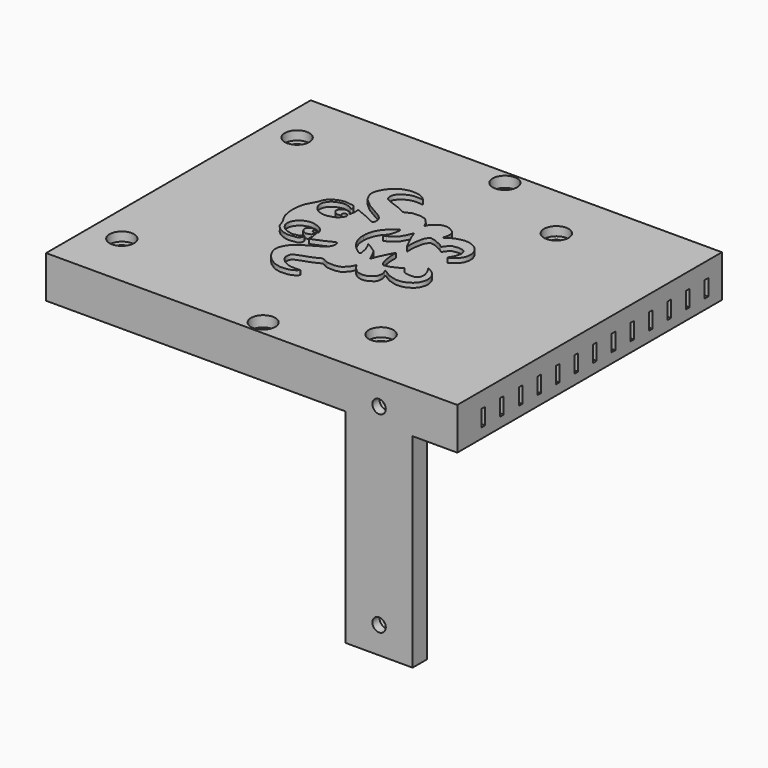
from build123d import *

# Parameters (mm, degrees)
F0_R      = 3
F0_R_2    = 1.45
F1_DEPTH  = 5
F2_W      = 88
F2_H      = 66
F3_DEPTH  = 3
F4_DEPTH  = 25
F5_R      = 2.75
F6_DEPTH  = 2
F7_W      = 7
F7_H      = 2
F8_DEPTH  = 9.4
F9_W      = 22.6646959782
F9_H      = 14.6112507209
F10_DEPTH = 2.9
F11_W     = 12
F11_H     = 4
F12_DEPTH = 5
F14_DEPTH = 1
F15_ANGLE = 90
F17_W     = 1
F17_H     = 3.667663259
F18_DEPTH = 5
F19_W     = 1
F19_H     = 3
F20_DEPTH = 2
F21_W     = 15
F21_H     = 45.6
F21_R     = 2.75
F21_H_2   = 9.4
F21_R_2   = 1.5
F22_DEPTH = 4
F23_DEPTH = 25
F24_START = -2
F24_DEPTH = 3
F25_R     = 1.7
F26_DEPTH = 25
F27_START = -7
F25_R_2   = 2.725
F27_DEPTH = 3


# Not quite as in the source:
# - ends of sketch curves that miss each other by under 0.0002 mm in the source are joined
# - a feature names something its author has since deleted; it is built from what else it names


with BuildPart() as f1:
    # F0 (on Top) → F1 (new body)
    with BuildSketch(Plane.XY):
        with Locations((-44.9419620109, 22.0892812656)):
            Circle(F0_R)
        with Locations((-44.9419620109, 22.0892812656)):
            Circle(F0_R_2, mode=Mode.SUBTRACT)
    extrude(amount=F1_DEPTH)



with BuildPart() as f1b:
    # F0 (on Top) → F1, piece 2 (new body)
    with BuildSketch(Plane.XY):
        with Locations((-44.9419620109, -26.9107187344)):
            Circle(F0_R)
        with Locations((-44.9419620109, -26.9107187344)):
            Circle(F0_R_2, mode=Mode.SUBTRACT)
    extrude(amount=F1_DEPTH)


with BuildPart() as f1c:
    # F0 (on Top) → F1, piece 3 (new body)
    with BuildSketch(Plane.XY):
        with Locations((13.0580379891, -26.9107187344)):
            Circle(F0_R)
        with Locations((13.0580379891, -26.9107187344)):
            Circle(F0_R_2, mode=Mode.SUBTRACT)
    extrude(amount=F1_DEPTH)


with BuildPart() as f1d:
    # F0 (on Top) → F1, piece 4 (new body)
    with BuildSketch(Plane.XY):
        with Locations((13.0580379891, 22.0892812656)):
            Circle(F0_R)
        with Locations((13.0580379891, 22.0892812656)):
            Circle(F0_R_2, mode=Mode.SUBTRACT)
    extrude(amount=F1_DEPTH)


with BuildPart() as f1_1:
    add(f1.part)

    add(f1b.part)  # F3 merges F1b

    add(f1c.part)  # F3 merges F1c

    add(f1d.part)  # F3 merges F1d
    # F2 (on face) → F3 (join)
    with BuildSketch(Plane.XY.offset(5)):
        with Locations((-5.8924814165, -2.4107187344)):
            Rectangle(F2_W, F2_H)
    extrude(amount=F3_DEPTH)

    # F0 (on Top) → F4 (cut)
    with BuildSketch(Plane.XY):
        with Locations((-44.9419620109, 22.0892812656)):
            Circle(F0_R_2)
        with Locations((-44.9419620109, -26.9107187344)):
            Circle(F0_R_2)
        with Locations((13.0580379891, -26.9107187344)):
            Circle(F0_R_2)
        with Locations((13.0580379891, 22.0892812656)):
            Circle(F0_R_2)
    extrude(amount=F4_DEPTH, mode=Mode.SUBTRACT)

    # F5 (on face) → F6 (cut)
    with BuildSketch(Plane.XY.offset(8)):
        with Locations((-44.9419620109, 22.0892812656)):
            Circle(F5_R)
        with Locations((-44.9419620109, -26.9107187344)):
            Circle(F5_R)
        with Locations((13.0580379891, -26.9107187344)):
            Circle(F5_R)
        with Locations((13.0580379891, 22.0892812656)):
            Circle(F5_R)
    extrude(amount=-F6_DEPTH, mode=Mode.SUBTRACT)

    # F7 (on face) → F8 (join)
    with BuildSketch(Plane.XY.offset(8)):
        Polygon((-9.3924814165, -35.4107187344), (-49.8924814165, -35.4107187344), (-49.8924814165, -39.4107187344), (38.1075185835, -39.4107187344), (38.1075185835, -35.4107187344), (-2.3924814165, -35.4107187344), align=None)
        Polygon((-49.8924814165, -39.4107187344), (-49.8924814165, -35.4107187344), (-49.8924814165, 30.5892812656), (-51.8924814165, 30.5892812656), (-51.8924814165, -39.4107187344), align=None)
        Polygon((-51.8924814165, 30.5892812656), (-49.8924814165, 30.5892812656), (-9.3924814165, 30.5892812656), (-2.3924814165, 30.5892812656), (38.1075185835, 30.5892812656), (38.1075185835, 34.5892812656), (-51.8924814165, 34.5892812656), align=None)
        Polygon((38.1075185835, -35.4107187344), (38.1075185835, -39.4107187344), (40.1075185835, -39.4107187344), (40.1075185835, 34.5892812656), (38.1075185835, 34.5892812656), (38.1075185835, 30.5892812656), align=None)
        with Locations((-5.8924814165, 29.5892812656)):
            Rectangle(F7_W, F7_H)
        with Locations((-5.8924814165, -34.4107187344)):
            Rectangle(F7_W, F7_H)
    extrude(amount=-F8_DEPTH)

    # F9 (on face) → F10 (cut)
    with BuildSketch(Plane(origin=(-51.8924814165, 0, 0), x_dir=(0, -1, 0), z_dir=(-1, 0, 0))):
        with Locations((-1.3754460961, -3.9222459309)):
            Rectangle(F9_W, F9_H)
    extrude(amount=-F10_DEPTH, mode=Mode.SUBTRACT)

    # F11 (on face) → F12 (cut)
    with BuildSketch(Plane(origin=(0, 34.5892812656, 0), x_dir=(-1, 0, 0), z_dir=(0, 1, 0))):
        with Locations((37.8924814165, 0.6)):
            Rectangle(F11_W, F11_H)
    extrude(amount=-F12_DEPTH, mode=Mode.SUBTRACT)

    # F17 (on face) → F18 (cut)
    with BuildSketch(Plane.YZ.offset(40.1075185835)):
        with Locations((-32.123142004, 2.647514717)):
            Rectangle(F17_W, F17_H)
        with Locations((-26.923142004, 2.647514717)):
            Rectangle(F17_W, F17_H)
        with Locations((-21.723142004, 2.647514717)):
            Rectangle(F17_W, F17_H)
        with Locations((-16.523142004, 2.647514717)):
            Rectangle(F17_W, F17_H)
        with Locations((-11.323142004, 2.647514717)):
            Rectangle(F17_W, F17_H)
        with Locations((-6.123142004, 2.647514717)):
            Rectangle(F17_W, F17_H)
        with Locations((-0.923142004, 2.647514717)):
            Rectangle(F17_W, F17_H)
        with Locations((4.276857996, 2.647514717)):
            Rectangle(F17_W, F17_H)
        with Locations((9.476857996, 2.647514717)):
            Rectangle(F17_W, F17_H)
        with Locations((14.676857996, 2.647514717)):
            Rectangle(F17_W, F17_H)
        with Locations((19.876857996, 2.647514717)):
            Rectangle(F17_W, F17_H)
        with Locations((25.076857996, 2.647514717)):
            Rectangle(F17_W, F17_H)
        with Locations((30.276857996, 2.647514717)):
            Rectangle(F17_W, F17_H)
    extrude(amount=-F18_DEPTH, mode=Mode.SUBTRACT)

    # F19 (on face) → F20 (cut)
    with BuildSketch(Plane(origin=(-51.8924814165, 0, 0), x_dir=(0, -1, 0), z_dir=(-1, 0, 0))):
        with Locations((-29.5138944983, 2.8654248323)):
            Rectangle(F19_W, F19_H)
        with Locations((-24.8138944983, 2.8654248323)):
            Rectangle(F19_W, F19_H)
        with Locations((-20.1138944983, 2.8654248323)):
            Rectangle(F19_W, F19_H)
        with Locations((-15.4138944983, 2.8654248323)):
            Rectangle(F19_W, F19_H)
        with Locations((12.1518093273, 2.8654248323)):
            Rectangle(F19_W, F19_H)
        with Locations((16.8518093273, 2.8654248323)):
            Rectangle(F19_W, F19_H)
        with Locations((21.5518093273, 2.8654248323)):
            Rectangle(F19_W, F19_H)
        with Locations((26.2518093273, 2.8654248323)):
            Rectangle(F19_W, F19_H)
        with Locations((30.9518093273, 2.8654248323)):
            Rectangle(F19_W, F19_H)
    extrude(amount=-F20_DEPTH, mode=Mode.SUBTRACT)



with BuildPart() as f14:
    # F13 (on face) → F14 (new body)
    with BuildSketch(Plane.XY.offset(8)):
        with BuildLine():
            add(Edge.make_bspline(
                [(11.5027878788, -2.4209789669), (11.7323937749, -2.6133507403), (12.0243123979, -2.9970076758), (12.3280450894, -3.5946591922), (12.5524157264, -4.3772097838), (12.5259593111, -5.2512184202), (12.6584274237, -5.9160082243), (12.3459932078, -6.7454326027), (12.2907721409, -7.3419620345), (11.8227509317, -7.9912359062), (11.4461462786, -8.6256120105), (10.9366706718, -9.1540031615), (10.279299862, -9.7593186059), (9.3011504467, -10.3201272531), (8.3010497276, -10.7813652421), (6.9906446073, -10.7385155761), (6.1121155177, -10.2690698993), (5.2420017435, -9.8082738598), (4.6879650789, -9.0157617746), (3.7801380878, -8.071640564), (3.436535335, -7.3101641754), (1.807130332, -4.4946267259), (1.4041576566, -4.1702507106), (1.0216456335, -3.7651965864), (0.530092257, -3.6391384278), (-0.0349250374, -3.5021356674), (-0.3309153572, -3.5574127738), (-0.8204993804, -3.6543530655), (-0.745590687, -4.1380303844), (-0.5788069953, -4.3625746728), (0.8008406604, -7.3625060277), (0.9305670164, -7.9599088855), (1.3857949569, -8.7091988221), (0.5230037317, -8.574928252), (0.1038875402, -8.4944949908), (-0.5011212843, -8.7803309715), (-0.9737544393, -8.6332500417), (-0.7821342736, -9.0808470613), (-0.4260377309, -9.1659516437), (-0.2778245709, -9.4533290208), (-0.1692147742, -9.7498501165), (-0.0414106572, -10.2621313495), (-0.1751833322, -10.5614539208), (-0.3589163113, -10.9501199194), (-0.6113378944, -11.2740165554), (-1.0948514105, -11.5278241366), (-1.4589498672, -11.5186409474), (-1.7749879439, -11.3714856649), (-1.9878530648, -11.0839489548), (-2.271933828, -10.8273821555), (-2.3617195813, -10.3632316908), (-2.3684991021, -10.1310438131), (-2.3552893082, -9.9029300604), (-2.2850273806, -9.3994208871), (-1.928311443, -9.9436267669), (-1.5979728154, -9.8953679473), (-1.3699771154, -9.7268378042), (-1.1952205318, -9.4219444501), (-1.2801187704, -9.0975929925), (-1.4508626111, -8.8270358173), (-1.8207786254, -8.6988880628), (-2.1294696426, -8.7408025919), (-2.8518412087, -9.2436090645), (-3.465126317, -9.9371351417), (-3.7421793211, -10.9199154012), (-3.9617364309, -11.7489927911), (-3.9108295177, -12.6684342258), (-3.6680667556, -13.2794532576), (-3.514746016, -13.811705088), (-3.0754026762, -14.2589619417), (-2.6280695922, -14.7186897696), (-2.0492313364, -15.0576497402), (-1.5264419438, -15.1857962636), (-0.8592645302, -15.246986214), (-0.2276608642, -15.0470096234), (0.5419057745, -14.5271446869), (0.9832770932, -13.8813790531), (1.3014524592, -13.2341913117), (1.4160235775, -12.6098139652), (1.6048664541, -11.9715718922), (1.3656048791, -11.0644805642), (1.3191050433, -10.5752118077), (0.3756103058, -9.5718079105), (2.0928065666, -9.9767744679), (2.0394706854, -10.8627502239), (2.1760345446, -11.4158707583), (2.2760377371, -12.254329737), (2.1835947978, -12.9610855254), (1.8830115129, -13.932006434), (1.3429782297, -14.8930222825), (0.3475643195, -15.8236109387), (-0.7338287183, -15.9725909006), (-1.9188408017, -16.7357698003), (-2.4507903803, -16.9718427751), (-2.9843508689, -17.3057685101), (-4.0131723225, -17.5156467898), (-5.0270536538, -17.6452261503), (-5.2578661318, -17.6894495777), (-5.74116024, -17.6808383201)],
                knots=[0, 0, 0, 0, 0.0113278181, 0.0216564788, 0.0331736661, 0.0450763538, 0.0556065125, 0.0673831726, 0.0773067991, 0.0885377298, 0.0995919188, 0.1104373121, 0.1225068946, 0.1360604283, 0.1495292594, 0.1638468047, 0.1766344186, 0.1890441223, 0.2017419474, 0.2158183599, 0.2285269993, 0.2512391435, 0.260808997, 0.2697448559, 0.2789832451, 0.2885583133, 0.2958142023, 0.3040244805, 0.3116755222, 0.3191619489, 0.3419644554, 0.3536291005, 0.3629190117, 0.372768302, 0.3817420852, 0.3921129509, 0.3994333427, 0.4064982536, 0.4142422024, 0.4211305296, 0.4284963449, 0.4375822723, 0.4448584175, 0.4531157234, 0.4613819201, 0.4706531962, 0.4782654692, 0.4855989067, 0.4931680578, 0.5010877694, 0.5097079586, 0.5157889165, 0.522313977, 0.5294262254, 0.5378668577, 0.5449124882, 0.5516346382, 0.5589584443, 0.5661544229, 0.5732980093, 0.5809471855, 0.5878994045, 0.5996382495, 0.6121208572, 0.62487722, 0.636835664, 0.648960899, 0.659313241, 0.6686668438, 0.6786542405, 0.6890029368, 0.6993417133, 0.7087448255, 0.7190110489, 0.7294035869, 0.7416082934, 0.7529683363, 0.7637373226, 0.773825986, 0.784268201, 0.7962812255, 0.8061074403, 0.8175060048, 0.830551438, 0.8419255087, 0.8517206106, 0.8632582146, 0.8741365549, 0.8868471812, 0.9004341261, 0.9149329378, 0.9284214137, 0.9433930736, 0.9531230049, 0.9629705281, 0.9762710491, 0.9884975027, 0.9999872829, 0.9999872829, 0.9999872829, 0.9999872829], degree=3))
            add(Edge.make_bspline(
                [(11.5027878788, -2.4209789669), (11.4401964379, -2.3407256192), (11.2716972898, -2.1246797747), (11.4317866708, -2.9475004184), (11.3781542644, -3.4708784631), (11.4308789187, -4.1304287661), (11.2856398352, -4.8860688558), (10.9730521948, -5.6732176246), (10.6086966376, -6.3246929617), (10.1015285444, -6.8583651375), (9.6338079197, -7.2731223467), (9.0388323784, -7.4959999547), (8.4935093686, -7.4653436969), (7.9465947831, -7.3810829532), (7.5963667745, -6.9987409993), (7.1714807695, -6.3481728764), (6.2781448691, -3.3191048874), (5.4129624132, -2.0816920073), (5.5609294619, -1.7811119332), (5.7984704652, -1.1768824975), (6.2419702832, -0.5540515495), (6.2150117261, 0.5485995398), (6.2768034692, 1.1067588451), (6.2082648196, 1.5211944169), (6.1198904153, 1.8680444073), (6.0419568813, 2.3385748282), (5.8432342897, 2.6134606762), (5.5408092745, 3.0124056346), (4.9276327602, 3.5628189122), (4.5123716459, 3.8845650329), (3.4123890719, 4.1779396414), (4.3402562294, 4.5098376645), (4.7242931928, 4.7738097714), (5.0435682073, 5.1545560799), (5.5351628785, 5.7313349538), (5.7262503452, 6.1215452397), (5.9049343311, 6.6491784829), (5.9852758802, 7.3003878263), (5.8520430596, 8.0873054068), (5.5136581046, 8.590955096), (5.154647, 9.2748249982), (4.7226400835, 9.5686592104), (4.3064267869, 9.6731543988), (3.6849899647, 9.8103311301), (3.1418185106, 9.6724271), (2.792299194, 9.6170814439), (2.0709391889, 9.2501622918), (2.6463999408, 10.1214556087), (2.9662825267, 10.6154197804), (3.266448923, 11.1236154517), (3.4682971053, 11.7655807641), (3.6387763469, 12.4247997992), (3.7799936238, 12.9662824833), (3.7742203546, 13.8649551622), (3.5994540219, 14.7162676312), (3.2858882988, 15.3298996316), (2.976434719, 15.8842313605), (2.6532966324, 16.3049551618), (1.9337663673, 16.9076911615), (1.3080502937, 17.0906117828), (0.8617865, 17.2921080104), (0.2737255646, 17.3221564076), (-0.3760939273, 17.2826142617), (-1.1219798958, 17.0796943827), (-1.6581268496, 16.748366985), (-2.215881576, 16.3239163979), (-2.5575477418, 15.7828498013), (-2.7947127653, 15.4133096102), (-3.3691922974, 14.5400247849), (-2.4315102387, 15.2017946951), (-1.8347899227, 15.4804262754), (-1.4047690674, 15.6121710386), (-0.7249667923, 15.8461276443), (-0.3178698123, 15.7882740082), (0.191021772, 15.7302157182), (0.4433920121, 15.5882639324), (0.7375296684, 15.2913697801), (0.9486923416, 14.8015956623), (0.9735477121, 14.3070506122), (1.02698231, 13.8462182885), (0.8667066144, 13.2920727109), (0.8569824924, 12.7357597584), (0.5561252691, 12.3803902807), (0.0601179723, 11.9087855377), (-0.358090528, 11.603797694), (-0.7777039608, 11.4148798548), (-0.1991945107, 10.8999674164), (0.050531353, 10.3611969011), (0.3735681453, 9.6778546323), (0.6891363028, 9.0368766401), (0.7409421366, 8.4052081477), (0.9340915725, 7.8754452799), (0.4825312523, 7.5059893845), (-0.0337378444, 7.1596737272), (-0.6295238881, 7.0091127836), (-1.279366567, 6.9254047366), (-1.707323154, 6.7949705556), (-3.2739097776, 6.616731026), (-4.5425710812, 6.8180780891), (-3.4053579094, 6.1923486801), (-2.7675522239, 5.975739096), (-1.8713257627, 5.4347509799), (-1.1024093736, 5.1005436845), (-0.3904107203, 4.866066957), (0.1014798295, 4.6746811095), (0.6431549197, 4.4980795385), (-0.645741324, 4.131973498), (-1.1569522903, 3.7579269143), (-1.9544752499, 3.4140863849), (-2.3643633804, 3.0596499008), (-2.7229806809, 2.4645410647), (-3.1022174791, 1.9145623998), (-3.3404859457, 1.5851150288), (-3.4565650176, 1.4264203912)],
                knots=[0, 0, 0, 0, 0.0051641522, 0.0138938833, 0.022805735, 0.0318062515, 0.0417720809, 0.052219875, 0.0620362989, 0.0717063449, 0.0806761406, 0.0895315344, 0.0979393094, 0.106192911, 0.1138430646, 0.1237389204, 0.1442427968, 0.1577186832, 0.1634575528, 0.1723631367, 0.1824143354, 0.1941674498, 0.2027533925, 0.2098653101, 0.2167360697, 0.2244463592, 0.2309468221, 0.2389710634, 0.2491029263, 0.2581405605, 0.2678251014, 0.2766350513, 0.28488036, 0.2928190882, 0.302636478, 0.310171599, 0.3184531895, 0.3277261924, 0.3376843233, 0.3466226782, 0.3565026495, 0.3644926525, 0.3718806117, 0.3809031065, 0.3892063419, 0.396562823, 0.4043162552, 0.4136473641, 0.4231238522, 0.4316232789, 0.4409648578, 0.4502701967, 0.4587462652, 0.4694329891, 0.4800715026, 0.489488084, 0.4983540247, 0.506689064, 0.5175784083, 0.5267585906, 0.5345656376, 0.5431259276, 0.5523702132, 0.5622583568, 0.5712971594, 0.5807666292, 0.5895889325, 0.5979282731, 0.6068149662, 0.6163733775, 0.6262361757, 0.633842416, 0.6432553581, 0.6507034669, 0.6586343202, 0.6646821125, 0.6718632104, 0.6801217769, 0.6880812868, 0.6957481137, 0.7043631541, 0.7126504308, 0.7202279335, 0.7296297968, 0.7380855981, 0.7442732711, 0.7530600301, 0.7622105066, 0.7720072375, 0.7816095224, 0.7906779926, 0.7986374764, 0.8067209667, 0.8157390832, 0.8247092912, 0.8336265471, 0.8412821177, 0.8561142691, 0.8660575812, 0.8761800375, 0.8864196507, 0.8977855677, 0.9083260546, 0.9180717772, 0.92673802, 0.9326065841, 0.9439193868, 0.9539633924, 0.9641722311, 0.9725255187, 0.9818749084, 0.9912242838, 1, 1, 1, 1], degree=3))
            add(Edge.make_bspline(
                [(-3.4565650176, 1.4264203912), (-3.6125875258, 1.1513369169), (-3.8879179466, 0.6659015166), (-3.3399356511, 1.041572901), (-3.1471047223, 1.1575660716), (-2.6874543722, 1.3348119514), (-2.3918531086, 1.4785638292), (-2.0367683679, 1.61498606), (-1.5410649966, 1.7357070754), (-1.0185296391, 1.8388000547), (-0.728742249, 1.8988747382), (-0.4258325496, 1.9192046951), (-0.2452958587, 1.9344673916), (0.0062209501, 1.7573060434), (-0.2486980208, 1.4051561564), (-0.5675214976, 0.9951983991), (-0.7745344154, 0.6725413955), (-1.1902945979, 0.2237398033), (-1.481073822, -0.0973922559), (-2.1700311939, -0.7598661256), (-2.805197493, -1.0745804528), (-3.4440837038, -1.4638527426), (-4.2494257854, -1.6818650964), (-4.9703995092, -1.8700028092), (-5.477510697, -1.8619258204), (-5.7419630446, -1.859926402)],
                knots=[0, 0, 0, 0, 0.049808879, 0.0880251541, 0.1215199585, 0.1642010424, 0.2006606201, 0.2385437689, 0.2838572942, 0.329472458, 0.3638952842, 0.3976216393, 0.4245081559, 0.4539181085, 0.4917629886, 0.5376282768, 0.577045643, 0.6246596122, 0.6671215712, 0.7272713167, 0.7807305651, 0.8342868672, 0.8913076689, 0.9452150642, 1, 1, 1, 1], degree=3))
            Line((-5.7419630446, -1.859926402), (-5.7419630446, -17.6808239944))
            add(Edge.make_bspline(
                [(-5.74116024, -17.6808383201), (-5.7414277277, -17.6808335541), (-5.7416953292, -17.6808287788), (-5.7419630446, -17.6808239944)],
                knots=[0.9999872829, 0.9999872829, 0.9999872829, 0.9999872829, 0.9999936421, 0.9999936421, 0.9999936421, 0.9999936421], degree=3))
        make_face()
        with BuildLine():
            add(Edge.make_bspline(
                [(-5.7419630446, -17.6808239944), (-5.7422307027, -17.6808192109), (-5.7424984747, -17.6808144183), (-5.7427663606, -17.6808096164)],
                knots=[0.9999936421, 0.9999936421, 0.9999936421, 0.9999936421, 1, 1, 1, 1], degree=3))
            Line((-5.7419630446, -17.6808239944), (-5.7419630446, -1.859926402))
            add(Edge.make_bspline(
                [(-8.0273610715, 1.4264203912), (-7.8713385633, 1.1513369169), (-7.5960081425, 0.6659015166), (-8.143990438, 1.041572901), (-8.3368213668, 1.1575660716), (-8.7964717169, 1.3348119514), (-9.0920729805, 1.4785638292), (-9.4471577212, 1.61498606), (-9.9428610925, 1.7357070754), (-10.46539645, 1.8388000547), (-10.7551838401, 1.8988747382), (-11.0580935395, 1.9192046951), (-11.2386302305, 1.9344673916), (-11.4901470392, 1.7573060434), (-11.2352280683, 1.4051561564), (-10.9164045915, 0.9951983991), (-10.7093916738, 0.6725413955), (-10.2936314912, 0.2237398033), (-10.0028522671, -0.0973922559), (-9.3138948952, -0.7598661256), (-8.6787285961, -1.0745804528), (-8.0398423853, -1.4638527426), (-7.2345003037, -1.6818650964), (-6.5135265799, -1.8700028092), (-6.0064153922, -1.8619258204), (-5.7419630446, -1.859926402)],
                knots=[0, 0, 0, 0, 0.049808879, 0.0880251541, 0.1215199585, 0.1642010424, 0.2006606201, 0.2385437689, 0.2838572942, 0.329472458, 0.3638952842, 0.3976216393, 0.4245081559, 0.4539181085, 0.4917629886, 0.5376282768, 0.577045643, 0.6246596122, 0.6671215712, 0.7272713167, 0.7807305651, 0.8342868672, 0.8913076689, 0.9452150642, 1, 1, 1, 1], degree=3))
            add(Edge.make_bspline(
                [(-22.9867139679, -2.4209789669), (-22.924122527, -2.3407256192), (-22.755623379, -2.1246797747), (-22.91571276, -2.9475004184), (-22.8620803535, -3.4708784631), (-22.9148050078, -4.1304287661), (-22.7695659243, -4.8860688558), (-22.456978284, -5.6732176246), (-22.0926227267, -6.3246929617), (-21.5854546335, -6.8583651375), (-21.1177340088, -7.2731223467), (-20.5227584676, -7.4959999547), (-19.9774354578, -7.4653436969), (-19.4305208722, -7.3810829532), (-19.0802928636, -6.9987409993), (-18.6554068586, -6.3481728764), (-17.7620709582, -3.3191048874), (-16.8968885023, -2.0816920073), (-17.044855551, -1.7811119332), (-17.2823965544, -1.1768824975), (-17.7258963723, -0.5540515495), (-17.6989378152, 0.5485995398), (-17.7607295583, 1.1067588451), (-17.6921909088, 1.5211944169), (-17.6038165044, 1.8680444073), (-17.5258829704, 2.3385748282), (-17.3271603788, 2.6134606762), (-17.0247353636, 3.0124056346), (-16.4115588493, 3.5628189122), (-15.996297735, 3.8845650329), (-14.8963151611, 4.1779396414), (-15.8241823185, 4.5098376645), (-16.2082192819, 4.7738097714), (-16.5274942964, 5.1545560799), (-17.0190889676, 5.7313349538), (-17.2101764343, 6.1215452397), (-17.3888604202, 6.6491784829), (-17.4692019693, 7.3003878263), (-17.3359691488, 8.0873054068), (-16.9975841937, 8.590955096), (-16.6385730892, 9.2748249982), (-16.2065661726, 9.5686592104), (-15.790352876, 9.6731543988), (-15.1689160538, 9.8103311301), (-14.6257445998, 9.6724271), (-14.2762252831, 9.6170814439), (-13.554865278, 9.2501622918), (-14.1303260299, 10.1214556087), (-14.4502086158, 10.6154197804), (-14.7503750122, 11.1236154517), (-14.9522231944, 11.7655807641), (-15.122702436, 12.4247997992), (-15.2639197129, 12.9662824833), (-15.2581464437, 13.8649551622), (-15.0833801111, 14.7162676312), (-14.7698143879, 15.3298996316), (-14.4603608081, 15.8842313605), (-14.1372227215, 16.3049551618), (-13.4176924564, 16.9076911615), (-12.7919763828, 17.0906117828), (-12.3457125892, 17.2921080104), (-11.7576516537, 17.3221564076), (-11.1078321618, 17.2826142617), (-10.3619461933, 17.0796943827), (-9.8257992395, 16.748366985), (-9.2680445131, 16.3239163979), (-8.9263783473, 15.7828498013), (-8.6892133239, 15.4133096102), (-8.1147337918, 14.5400247849), (-9.0524158504, 15.2017946951), (-9.6491361664, 15.4804262754), (-10.0791570217, 15.6121710386), (-10.7589592968, 15.8461276443), (-11.1660562768, 15.7882740082), (-11.6749478611, 15.7302157182), (-11.9273181012, 15.5882639324), (-12.2214557576, 15.2913697801), (-12.4326184308, 14.8015956623), (-12.4574738012, 14.3070506122), (-12.5109083991, 13.8462182885), (-12.3506327036, 13.2920727109), (-12.3409085815, 12.7357597584), (-12.0400513582, 12.3803902807), (-11.5440440614, 11.9087855377), (-11.1258355612, 11.603797694), (-10.7062221283, 11.4148798548), (-11.2847315784, 10.8999674164), (-11.5344574422, 10.3611969011), (-11.8574942344, 9.6778546323), (-12.1730623919, 9.0368766401), (-12.2248682257, 8.4052081477), (-12.4180176617, 7.8754452799), (-11.9664573414, 7.5059893845), (-11.4501882448, 7.1596737272), (-10.8544022011, 7.0091127836), (-10.2045595221, 6.9254047366), (-9.7766029351, 6.7949705556), (-8.2100163116, 6.616731026), (-6.9413550079, 6.8180780891), (-8.0785681798, 6.1923486801), (-8.7163738652, 5.975739096), (-9.6126003265, 5.4347509799), (-10.3815167155, 5.1005436845), (-11.0935153688, 4.866066957), (-11.5854059186, 4.6746811095), (-12.1270810089, 4.4980795385), (-10.8381847651, 4.131973498), (-10.3269737988, 3.7579269143), (-9.5294508392, 3.4140863849), (-9.1195627087, 3.0596499008), (-8.7609454082, 2.4645410647), (-8.38170861, 1.9145623998), (-8.1434401435, 1.5851150288), (-8.0273610715, 1.4264203912)],
                knots=[0, 0, 0, 0, 0.0051641522, 0.0138938833, 0.022805735, 0.0318062515, 0.0417720809, 0.052219875, 0.0620362989, 0.0717063449, 0.0806761406, 0.0895315344, 0.0979393094, 0.106192911, 0.1138430646, 0.1237389204, 0.1442427968, 0.1577186832, 0.1634575528, 0.1723631367, 0.1824143354, 0.1941674498, 0.2027533925, 0.2098653101, 0.2167360697, 0.2244463592, 0.2309468221, 0.2389710634, 0.2491029263, 0.2581405605, 0.2678251014, 0.2766350513, 0.28488036, 0.2928190882, 0.302636478, 0.310171599, 0.3184531895, 0.3277261924, 0.3376843233, 0.3466226782, 0.3565026495, 0.3644926525, 0.3718806117, 0.3809031065, 0.3892063419, 0.396562823, 0.4043162552, 0.4136473641, 0.4231238522, 0.4316232789, 0.4409648578, 0.4502701967, 0.4587462652, 0.4694329891, 0.4800715026, 0.489488084, 0.4983540247, 0.506689064, 0.5175784083, 0.5267585906, 0.5345656376, 0.5431259276, 0.5523702132, 0.5622583568, 0.5712971594, 0.5807666292, 0.5895889325, 0.5979282731, 0.6068149662, 0.6163733775, 0.6262361757, 0.633842416, 0.6432553581, 0.6507034669, 0.6586343202, 0.6646821125, 0.6718632104, 0.6801217769, 0.6880812868, 0.6957481137, 0.7043631541, 0.7126504308, 0.7202279335, 0.7296297968, 0.7380855981, 0.7442732711, 0.7530600301, 0.7622105066, 0.7720072375, 0.7816095224, 0.7906779926, 0.7986374764, 0.8067209667, 0.8157390832, 0.8247092912, 0.8336265471, 0.8412821177, 0.8561142691, 0.8660575812, 0.8761800375, 0.8864196507, 0.8977855677, 0.9083260546, 0.9180717772, 0.92673802, 0.9326065841, 0.9439193868, 0.9539633924, 0.9641722311, 0.9725255187, 0.9818749084, 0.9912242838, 1, 1, 1, 1], degree=3))
            add(Edge.make_bspline(
                [(-22.9867139679, -2.4209789669), (-23.216319864, -2.6133507403), (-23.5082384871, -2.9970076758), (-23.8119711786, -3.5946591922), (-24.0363418155, -4.3772097838), (-24.0098854002, -5.2512184202), (-24.1423535128, -5.9160082243), (-23.8299192969, -6.7454326027), (-23.77469823, -7.3419620345), (-23.3066770208, -7.9912359062), (-22.9300723677, -8.6256120105), (-22.420596761, -9.1540031615), (-21.7632259512, -9.7593186059), (-20.7850765358, -10.3201272531), (-19.7849758167, -10.7813652421), (-18.4745706964, -10.7385155761), (-17.5960416068, -10.2690698993), (-16.7259278326, -9.8082738598), (-16.1718911681, -9.0157617746), (-15.2640641769, -8.071640564), (-14.9204614242, -7.3101641754), (-13.2910564212, -4.4946267259), (-12.8880837457, -4.1702507106), (-12.5055717227, -3.7651965864), (-12.0140183462, -3.6391384278), (-11.4490010517, -3.5021356674), (-11.1530107319, -3.5574127738), (-10.6634267087, -3.6543530655), (-10.7383354022, -4.1380303844), (-10.9051190939, -4.3625746728), (-12.2847667495, -7.3625060277), (-12.4144931055, -7.9599088855), (-12.8697210461, -8.7091988221), (-12.0069298208, -8.574928252), (-11.5878136294, -8.4944949908), (-10.9828048048, -8.7803309715), (-10.5101716499, -8.6332500417), (-10.7017918155, -9.0808470613), (-11.0578883582, -9.1659516437), (-11.2061015182, -9.4533290208), (-11.314711315, -9.7498501165), (-11.4425154319, -10.2621313495), (-11.3087427569, -10.5614539208), (-11.1250097778, -10.9501199194), (-10.8725881948, -11.2740165554), (-10.3890746787, -11.5278241366), (-10.0249762219, -11.5186409474), (-9.7089381452, -11.3714856649), (-9.4960730243, -11.0839489548), (-9.2119922611, -10.8273821555), (-9.1222065078, -10.3632316908), (-9.115426987, -10.1310438131), (-9.1286367809, -9.9029300604), (-9.1988987085, -9.3994208871), (-9.5556146461, -9.9436267669), (-9.8859532737, -9.8953679473), (-10.1139489737, -9.7268378042), (-10.2887055573, -9.4219444501), (-10.2038073187, -9.0975929925), (-10.033063478, -8.8270358173), (-9.6631474638, -8.6988880628), (-9.3544564465, -8.7408025919), (-8.6320848804, -9.2436090645), (-8.0187997721, -9.9371351417), (-7.741746768, -10.9199154012), (-7.5221896582, -11.7489927911), (-7.5730965715, -12.6684342258), (-7.8158593335, -13.2794532576), (-7.9691800731, -13.811705088), (-8.4085234129, -14.2589619417), (-8.8558564969, -14.7186897696), (-9.4346947528, -15.0576497402), (-9.9574841453, -15.1857962636), (-10.6246615589, -15.246986214), (-11.2562652249, -15.0470096234), (-12.0258318636, -14.5271446869), (-12.4672031823, -13.8813790531), (-12.7853785483, -13.2341913117), (-12.8999496666, -12.6098139652), (-13.0887925432, -11.9715718922), (-12.8495309683, -11.0644805642), (-12.8030311324, -10.5752118077), (-11.8595363949, -9.5718079105), (-13.5767326557, -9.9767744679), (-13.5233967746, -10.8627502239), (-13.6599606338, -11.4158707583), (-13.7599638263, -12.254329737), (-13.6675208869, -12.9610855254), (-13.3669376021, -13.932006434), (-12.8269043188, -14.8930222825), (-11.8314904086, -15.8236109387), (-10.7500973709, -15.9725909006), (-9.5650852874, -16.7357698003), (-9.0331357088, -16.9718427751), (-8.4995752202, -17.3057685101), (-7.4707537666, -17.5156467898), (-6.4568724353, -17.6452261503), (-6.2260599573, -17.6894495777), (-5.7427663606, -17.6808096164)],
                knots=[0, 0, 0, 0, 0.0113278181, 0.0216564788, 0.0331736661, 0.0450763538, 0.0556065125, 0.0673831726, 0.0773067991, 0.0885377298, 0.0995919188, 0.1104373121, 0.1225068946, 0.1360604283, 0.1495292594, 0.1638468047, 0.1766344186, 0.1890441223, 0.2017419474, 0.2158183599, 0.2285269993, 0.2512391435, 0.260808997, 0.2697448559, 0.2789832451, 0.2885583133, 0.2958142023, 0.3040244805, 0.3116755222, 0.3191619489, 0.3419644554, 0.3536291005, 0.3629190117, 0.372768302, 0.3817420852, 0.3921129509, 0.3994333427, 0.4064982536, 0.4142422024, 0.4211305296, 0.4284963449, 0.4375822723, 0.4448584175, 0.4531157234, 0.4613819201, 0.4706531962, 0.4782654692, 0.4855989067, 0.4931680578, 0.5010877694, 0.5097079586, 0.5157889165, 0.522313977, 0.5294262254, 0.5378668577, 0.5449124882, 0.5516346382, 0.5589584443, 0.5661544229, 0.5732980093, 0.5809471855, 0.5878994045, 0.5996382495, 0.6121208572, 0.62487722, 0.636835664, 0.648960899, 0.659313241, 0.6686668438, 0.6786542405, 0.6890029368, 0.6993417133, 0.7087448255, 0.7190110489, 0.7294035869, 0.7416082934, 0.7529683363, 0.7637373226, 0.773825986, 0.784268201, 0.7962812255, 0.8061074403, 0.8175060048, 0.830551438, 0.8419255087, 0.8517206106, 0.8632582146, 0.8741365549, 0.8868471812, 0.9004341261, 0.9149329378, 0.9284214137, 0.9433930736, 0.9531230049, 0.9629705281, 0.9762710491, 0.9884975027, 0.9999872829, 0.9999872829, 0.9999872829, 0.9999872829], degree=3))
        make_face()
    extrude(amount=F14_DEPTH)


with BuildPart() as f14_1:
    # F15: moved
    add(f14.part.rotate(Axis((-3.4565650176, 1.4264203912, 8.5), (0, 0, -1)), F15_ANGLE))


with BuildPart() as f14_2:
    # F16: moved
    add(f14_1.part.moved(Location((-4.8, -4.8, 0))))


with BuildPart() as f1_2:
    add(f1_1.part)

    add(f14_2.part)  # F22 merges F14
    # F21 (on face) → F22 (join, through all)
    with BuildSketch(Plane.XZ.offset(39.4107187344)):
        with Locations((22.6075185835, -24.2)):
            Rectangle(F21_W, F21_H)
        with Locations((22.6075185835, -41)):
            Circle(F21_R, mode=Mode.SUBTRACT)
        with Locations((22.6075185835, 3.3)):
            Rectangle(F21_W, F21_H_2)
        with Locations((22.6075185835, 2)):
            Circle(F21_R, mode=Mode.SUBTRACT)
        with Locations((22.6075185835, -41)):
            Circle(F21_R)
        with Locations((22.6075185835, -41)):
            Circle(F21_R_2, mode=Mode.SUBTRACT)
    extrude(amount=-F22_DEPTH)

    # F21 (on face) → F23 (cut)
    with BuildSketch(Plane.XZ.offset(39.4107187344)):
        with Locations((22.6075185835, 2)):
            Circle(F21_R_2)
    extrude(amount=-F23_DEPTH, mode=Mode.SUBTRACT)

    # F21 (on face) → F24 (cut)
    with BuildSketch(Plane.XZ.offset(39.4107187344).offset(F24_START)):
        with Locations((22.6075185835, 2)):
            Circle(F21_R)
        with Locations((22.6075185835, 2)):
            Circle(F21_R_2, mode=Mode.SUBTRACT)
        with Locations((22.6075185835, -41)):
            Circle(F21_R)
        with Locations((22.6075185835, -41)):
            Circle(F21_R_2, mode=Mode.SUBTRACT)
    extrude(amount=-F24_DEPTH, mode=Mode.SUBTRACT)

    # F25 (on face) → F26 (cut)
    with BuildSketch(Plane(origin=(0, 0, -1.4), x_dir=(1, 0, 0), z_dir=(0, 0, -1))):
        with Locations((-5.8924814165, 36.2107187344)):
            Circle(F25_R)
        with Locations((-5.8924814165, -31.3892812656)):
            Circle(F25_R)
    extrude(amount=-F26_DEPTH, mode=Mode.SUBTRACT)

    # F25 (on face) → F27 (cut)
    with BuildSketch(Plane(origin=(0, 0, -1.4), x_dir=(1, 0, 0), z_dir=(0, 0, -1)).offset(F27_START)):
        with Locations((-5.8924814165, 36.2107187344)):
            Circle(F25_R_2)
        with Locations((-5.8924814165, 36.2107187344)):
            Circle(F25_R, mode=Mode.SUBTRACT)
        with Locations((-5.8924814165, -31.3892812656)):
            Circle(F25_R_2)
        with Locations((-5.8924814165, -31.3892812656)):
            Circle(F25_R, mode=Mode.SUBTRACT)
    extrude(amount=-F27_DEPTH, mode=Mode.SUBTRACT)


solid = f1_2.part
